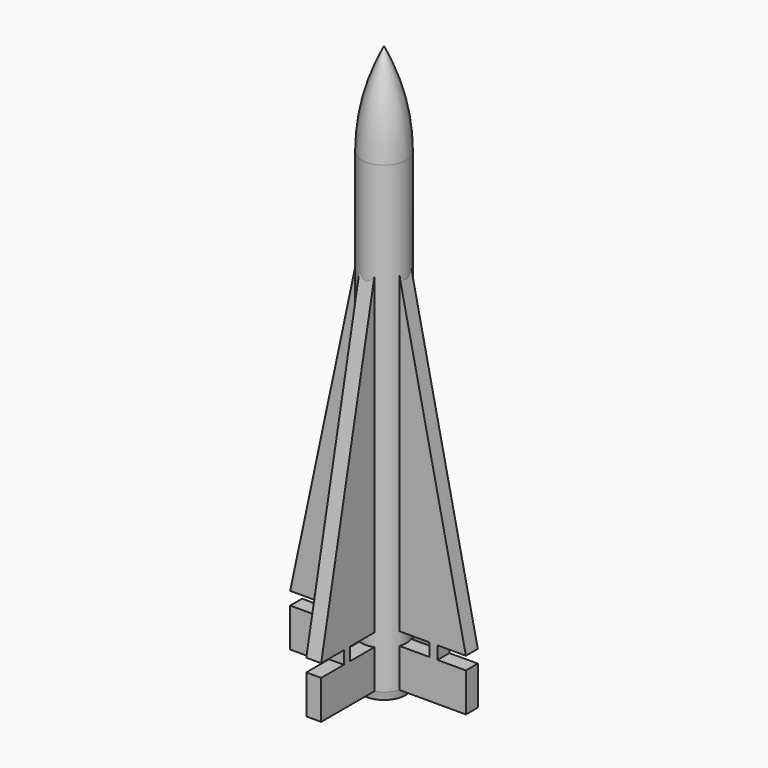
from build123d import *

# Parameters (mm, degrees)
F2_W     = 0.2083333333
F2_H     = 0.3472222222
F3_DEPTH = 0.2
F4_COUNT = 4


# Not quite as in the source:
# - a feature names something its author has since deleted; it is built from what else it names


with BuildPart() as f1:
    # F0 (on Front) → F1 (revolve)
    with BuildSketch(Plane.XZ):
        with BuildLine():
            Line((0, 15.1736111111), (0, 0))
            Line((0, 0), (0.5729166667, 0))
            Line((0.5729166667, 0), (0.6076388889, 0.2083333333))
            Line((0.6076388889, 0.2083333333), (0.6076388889, 12.6736111111))
            ThreePointArc((0.6076388889, 12.6736111111), (0.453549532, 13.9600038407), (0, 15.1736111111))
        make_face()
    revolve(axis=Axis((0, 0, 7.5868055556), (0, 0, 1)))

    # F2 (on Front) → F3 (join, symmetric)
    with BuildSketch(Plane.XZ):
        Polygon((0, 11.3755206646), (0, 0.2083333333), (0.6076388889, 0.2083333333), (2.3611111111, 0.2083333333), (2.3611111111, 1.25), (1.5972222222, 1.25), (1.3888888889, 1.25), (0.4, 1.25), (0.4, 1.5972222222), (1.3888888889, 1.5972222222), (1.5972222222, 1.5972222222), (2.3611111111, 1.5972222222), (0.2863040887, 11.3755206646), align=None)
        with Locations((1.4930555556, 1.4236111111)):
            Rectangle(F2_W, F2_H)
    extrude(amount=F3_DEPTH, both=True)

    # F4: F1 ×4 about axis
    f4_axis = Axis((0, 0, 0.2083333333), (0, 0, 1))


with BuildPart() as f1_1:
    add(f1.part)
    for i in range(1, F4_COUNT):
        add(f1.part.rotate(f4_axis, i * 360 / F4_COUNT))


solid = f1_1.part
